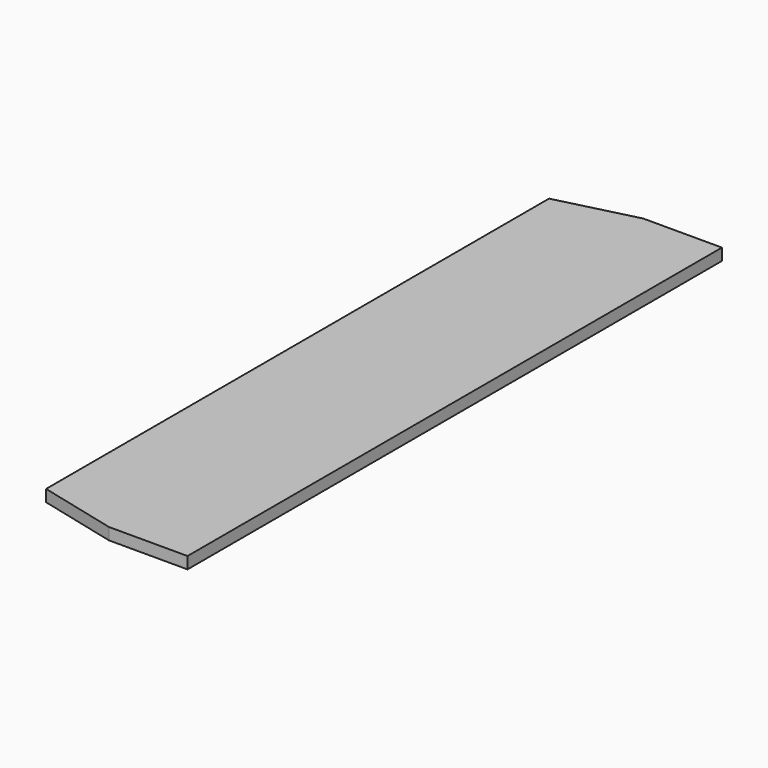
from build123d import *

# Parameters (mm, degrees)
F0_W     = 40
F0_H     = 170
F1_DEPTH = 3
F2_SIZE2 = 5
F2_SIZE  = 20
F3_SIZE2 = 20
F3_SIZE  = 5


with BuildPart() as f1:
    # F0 (on Top) → F1 (new body)
    with BuildSketch(Plane.XY):
        with Locations((-39.5484667792, 0.5357116461)):
            Rectangle(F0_W, F0_H)
    extrude(amount=F1_DEPTH)

    # F2
    f2_edges = [f1.edges().sort_by_distance(p)[0] for p in [
        (-59.548467, -84.464288, 1.5),
    ]]
    f2_side = f1.faces().sort_by_distance((-39.548467, -84.464288, 1.5))[0]
    chamfer(f2_edges, length=F2_SIZE, length2=F2_SIZE2, reference=f2_side)

    # F3
    f3_edges = [f1.edges().sort_by_distance(p)[0] for p in [
        (-59.548467, 85.535712, 1.5),
    ]]
    f3_side = f1.faces().sort_by_distance((-59.548467, 3.035712, 1.5))[0]
    chamfer(f3_edges, length=F3_SIZE, length2=F3_SIZE2, reference=f3_side)


solid = f1.part
